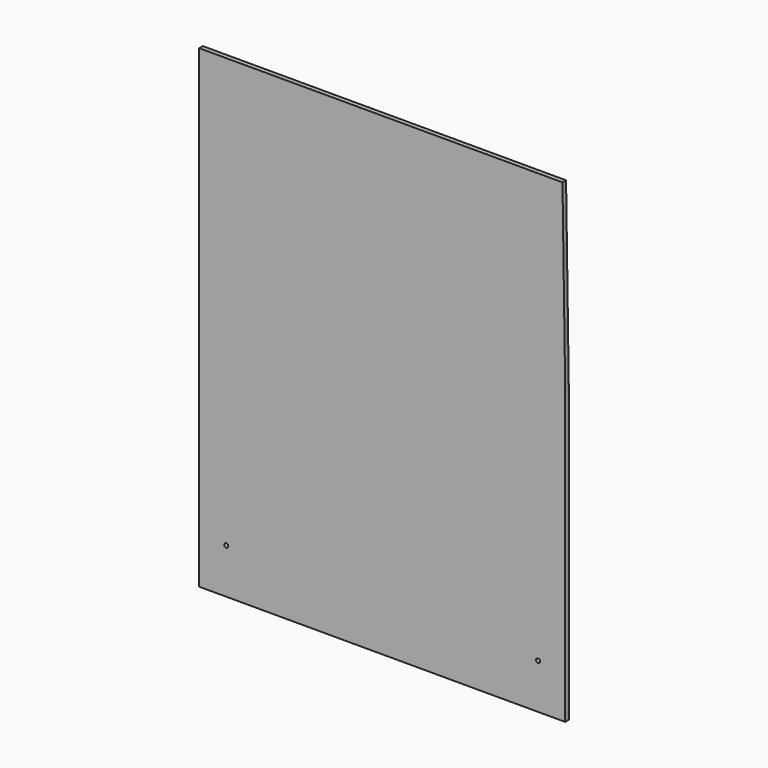
from build123d import *

# Parameters (mm, degrees)
F1_DEPTH = 5
F2_R     = 2.25
F3_DEPTH = 5


# Not quite as in the source:
# - a feature names something its author has since deleted; it is built from what else it names


with BuildPart() as f1:
    # F0 (on Front) → F1 (new body)
    with BuildSketch(Plane.XZ):
        Polygon((0, 526), (0, 0), (406, 0), (406, 326), (403, 526), align=None)
    extrude(amount=F1_DEPTH)

    # F2 (on face) → F3 (cut, through all)
    with BuildSketch(Plane.XZ.offset(5)):
        with Locations((30, 50)):
            Circle(F2_R)
        with Locations((376, 50)):
            Circle(F2_R)
    extrude(amount=-F3_DEPTH, mode=Mode.SUBTRACT)


solid = f1.part
